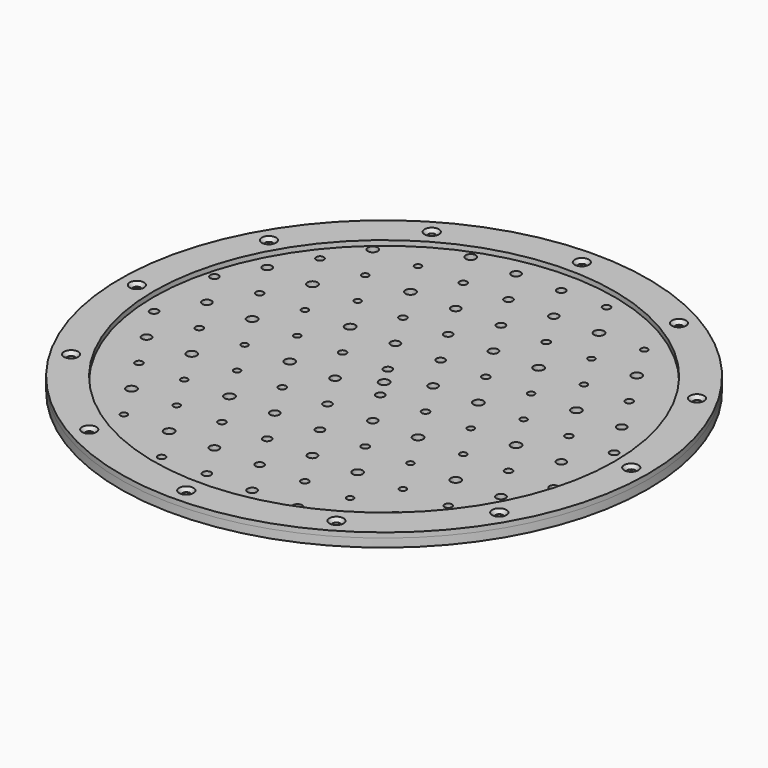
from build123d import *

# Parameters (mm, degrees)
F0_R     = 2.25
F0_R_2   = 2
F0_R_3   = 3
F0_R_4   = 2.75
F0_R_5   = 2.5
F1_DEPTH = 5
F2_R     = 157.5
F2_R_2   = 2
F2_R_3   = 137.5
F3_DEPTH = 5
F4_R     = 157.5
F4_R_2   = 2.25
F4_R_3   = 137.5
F5_DEPTH = 3
F6_SIZE  = 2


# Not quite as in the source:
# - a feature names something its author has since deleted; it is built from what else it names


with BuildPart() as f1:
    # F0 (on Top) → F1 (new body)
    with BuildSketch(Plane.XY):
        with BuildLine():
            Line((47.25, 82.8640606254), (47.25, 75.5725751183))
            ThreePointArc((47.25, 75.5725751183), (114.75, 57.8640606254), (182.25, 75.5725751183))
            ThreePointArc((182.25, 75.5725751183), (233.4671007058, 125.9918759979), (252.25, 195.3640606254))
            ThreePointArc((252.25, 195.3640606254), (233.4671007058, 264.736245253), (182.25, 315.1555461325))
            ThreePointArc((182.25, 315.1555461325), (114.75, 332.8640606254), (47.25, 315.1555461325))
            ThreePointArc((47.25, 315.1555461325), (-22.580141759, 202.1964953641), (35.6930584958, 82.8640606254))
            Line((35.6930584958, 82.8640606254), (47.25, 82.8640606254))
        make_face()
        with Locations((81, 71.6140606254)):
            Circle(F0_R, mode=Mode.SUBTRACT)
        with Locations((40.5, 94.1140606254)):
            Circle(F0_R_2, mode=Mode.SUBTRACT)
        with Locations((27, 116.6140606254)):
            Circle(F0_R_3, mode=Mode.SUBTRACT)
        with Locations((67.5, 94.1140606254)):
            Circle(F0_R_3, mode=Mode.SUBTRACT)
        with Locations((54, 116.6140606254)):
            Circle(F0_R_2, mode=Mode.SUBTRACT)
        with Locations((81, 116.6140606254)):
            Circle(F0_R, mode=Mode.SUBTRACT)
        with Locations((13.5, 139.1140606254)):
            Circle(F0_R, mode=Mode.SUBTRACT)
        with Locations((40.5, 139.1140606254)):
            Circle(F0_R_2, mode=Mode.SUBTRACT)
        with Locations((0, 161.6140606254)):
            Circle(F0_R_4, mode=Mode.SUBTRACT)
        with Locations((27, 161.6140606254)):
            Circle(F0_R_3, mode=Mode.SUBTRACT)
        with Locations((67.5, 139.1140606254)):
            Circle(F0_R_3, mode=Mode.SUBTRACT)
        with Locations((54, 161.6140606254)):
            Circle(F0_R_2, mode=Mode.SUBTRACT)
        with Locations((81, 161.6140606254)):
            Circle(F0_R, mode=Mode.SUBTRACT)
        with Locations((108, 71.6140606254)):
            Circle(F0_R_5, mode=Mode.SUBTRACT)
        with Locations((135, 71.6140606254)):
            Circle(F0_R_4, mode=Mode.SUBTRACT)
        with Locations((162, 71.6140606254)):
            Circle(F0_R_3, mode=Mode.SUBTRACT)
        with Locations((94.5, 94.1140606254)):
            Circle(F0_R_4, mode=Mode.SUBTRACT)
        with Locations((121.5, 94.1140606254)):
            Circle(F0_R_5, mode=Mode.SUBTRACT)
        with Locations((108, 116.6140606254)):
            Circle(F0_R_5, mode=Mode.SUBTRACT)
        with Locations((148.5, 94.1140606254)):
            Circle(F0_R, mode=Mode.SUBTRACT)
        with Locations((135, 116.6140606254)):
            Circle(F0_R_4, mode=Mode.SUBTRACT)
        with Locations((162, 116.6140606254)):
            Circle(F0_R_3, mode=Mode.SUBTRACT)
        with Locations((94.5, 139.1140606254)):
            Circle(F0_R_4, mode=Mode.SUBTRACT)
        with Locations((121.5, 139.1140606254)):
            Circle(F0_R_5, mode=Mode.SUBTRACT)
        with Locations((108, 161.6140606254)):
            Circle(F0_R_5, mode=Mode.SUBTRACT)
        with Locations((148.5, 139.1140606254)):
            Circle(F0_R, mode=Mode.SUBTRACT)
        with Locations((135, 161.6140606254)):
            Circle(F0_R_4, mode=Mode.SUBTRACT)
        with Locations((162, 161.6140606254)):
            Circle(F0_R_3, mode=Mode.SUBTRACT)
        with Locations((175.5, 94.1140606254)):
            Circle(F0_R_2, mode=Mode.SUBTRACT)
        with Locations((202.5, 94.1140606254)):
            Circle(F0_R_3, mode=Mode.SUBTRACT)
        with Locations((189, 116.6140606254)):
            Circle(F0_R_2, mode=Mode.SUBTRACT)
        with Locations((216, 116.6140606254)):
            Circle(F0_R, mode=Mode.SUBTRACT)
        with Locations((175.5, 139.1140606254)):
            Circle(F0_R_2, mode=Mode.SUBTRACT)
        with Locations((202.5, 139.1140606254)):
            Circle(F0_R_3, mode=Mode.SUBTRACT)
        with Locations((189, 161.6140606254)):
            Circle(F0_R_2, mode=Mode.SUBTRACT)
        with Locations((229.5, 139.1140606254)):
            Circle(F0_R_4, mode=Mode.SUBTRACT)
        with Locations((216, 161.6140606254)):
            Circle(F0_R, mode=Mode.SUBTRACT)
        with Locations((243, 161.6140606254)):
            Circle(F0_R_5, mode=Mode.SUBTRACT)
        with Locations((-13.5, 184.1140606254)):
            Circle(F0_R_5, mode=Mode.SUBTRACT)
        with Locations((-13.5, 229.1140606254)):
            Circle(F0_R_5, mode=Mode.SUBTRACT)
        with Locations((13.5, 184.1140606254)):
            Circle(F0_R, mode=Mode.SUBTRACT)
        with Locations((40.5, 184.1140606254)):
            Circle(F0_R_2, mode=Mode.SUBTRACT)
        with Locations((0, 206.6140606254)):
            Circle(F0_R_4, mode=Mode.SUBTRACT)
        with Locations((27, 206.6140606254)):
            Circle(F0_R_3, mode=Mode.SUBTRACT)
        with Locations((67.5, 184.1140606254)):
            Circle(F0_R_3, mode=Mode.SUBTRACT)
        with Locations((54, 206.6140606254)):
            Circle(F0_R_2, mode=Mode.SUBTRACT)
        with Locations((81, 206.6140606254)):
            Circle(F0_R, mode=Mode.SUBTRACT)
        with Locations((13.5, 229.1140606254)):
            Circle(F0_R, mode=Mode.SUBTRACT)
        with Locations((40.5, 229.1140606254)):
            Circle(F0_R_2, mode=Mode.SUBTRACT)
        with Locations((0, 251.6140606254)):
            Circle(F0_R_4, mode=Mode.SUBTRACT)
        with Locations((27, 251.6140606254)):
            Circle(F0_R_3, mode=Mode.SUBTRACT)
        with Locations((67.5, 229.1140606254)):
            Circle(F0_R_3, mode=Mode.SUBTRACT)
        with Locations((54, 251.6140606254)):
            Circle(F0_R_2, mode=Mode.SUBTRACT)
        with Locations((81, 251.6140606254)):
            Circle(F0_R, mode=Mode.SUBTRACT)
        with Locations((13.5, 274.1140606254)):
            Circle(F0_R, mode=Mode.SUBTRACT)
        with Locations((40.5, 274.1140606254)):
            Circle(F0_R_2, mode=Mode.SUBTRACT)
        with Locations((27, 296.6140606254)):
            Circle(F0_R_3, mode=Mode.SUBTRACT)
        with Locations((67.5, 274.1140606254)):
            Circle(F0_R_3, mode=Mode.SUBTRACT)
        with Locations((54, 296.6140606254)):
            Circle(F0_R_2, mode=Mode.SUBTRACT)
        with Locations((81, 296.6140606254)):
            Circle(F0_R, mode=Mode.SUBTRACT)
        with Locations((67.5, 319.1140606254)):
            Circle(F0_R_3, mode=Mode.SUBTRACT)
        with Locations((94.5, 184.1140606254)):
            Circle(F0_R_4, mode=Mode.SUBTRACT)
        with Locations((121.5, 184.1140606254)):
            Circle(F0_R_5, mode=Mode.SUBTRACT)
        with Locations((114.8160025477, 195.3414678574)):
            Circle(F0_R_3, mode=Mode.SUBTRACT)
        with Locations((108, 206.6140606254)):
            Circle(F0_R_5, mode=Mode.SUBTRACT)
        with Locations((148.5, 184.1140606254)):
            Circle(F0_R, mode=Mode.SUBTRACT)
        with Locations((135, 206.6140606254)):
            Circle(F0_R_4, mode=Mode.SUBTRACT)
        with Locations((162, 206.6140606254)):
            Circle(F0_R_3, mode=Mode.SUBTRACT)
        with Locations((94.5, 229.1140606254)):
            Circle(F0_R_4, mode=Mode.SUBTRACT)
        with Locations((121.5, 229.1140606254)):
            Circle(F0_R_5, mode=Mode.SUBTRACT)
        with Locations((108, 251.6140606254)):
            Circle(F0_R_5, mode=Mode.SUBTRACT)
        with Locations((148.5, 229.1140606254)):
            Circle(F0_R, mode=Mode.SUBTRACT)
        with Locations((135, 251.6140606254)):
            Circle(F0_R_4, mode=Mode.SUBTRACT)
        with Locations((162, 251.6140606254)):
            Circle(F0_R_3, mode=Mode.SUBTRACT)
        with Locations((175.5, 184.1140606254)):
            Circle(F0_R_2, mode=Mode.SUBTRACT)
        with Locations((202.5, 184.1140606254)):
            Circle(F0_R_3, mode=Mode.SUBTRACT)
        with Locations((189, 206.6140606254)):
            Circle(F0_R_2, mode=Mode.SUBTRACT)
        with Locations((229.5, 184.1140606254)):
            Circle(F0_R_4, mode=Mode.SUBTRACT)
        with Locations((216, 206.6140606254)):
            Circle(F0_R, mode=Mode.SUBTRACT)
        with Locations((243, 206.6140606254)):
            Circle(F0_R_5, mode=Mode.SUBTRACT)
        with Locations((175.5, 229.1140606254)):
            Circle(F0_R_2, mode=Mode.SUBTRACT)
        with Locations((202.5, 229.1140606254)):
            Circle(F0_R_3, mode=Mode.SUBTRACT)
        with Locations((189, 251.6140606254)):
            Circle(F0_R_2, mode=Mode.SUBTRACT)
        with Locations((229.5, 229.1140606254)):
            Circle(F0_R_4, mode=Mode.SUBTRACT)
        with Locations((216, 251.6140606254)):
            Circle(F0_R, mode=Mode.SUBTRACT)
        with Locations((94.5, 274.1140606254)):
            Circle(F0_R_4, mode=Mode.SUBTRACT)
        with Locations((121.5, 274.1140606254)):
            Circle(F0_R_5, mode=Mode.SUBTRACT)
        with Locations((108, 296.6140606254)):
            Circle(F0_R_5, mode=Mode.SUBTRACT)
        with Locations((148.5, 274.1140606254)):
            Circle(F0_R, mode=Mode.SUBTRACT)
        with Locations((135, 296.6140606254)):
            Circle(F0_R_4, mode=Mode.SUBTRACT)
        with Locations((162, 296.6140606254)):
            Circle(F0_R_3, mode=Mode.SUBTRACT)
        with Locations((94.5, 319.1140606254)):
            Circle(F0_R_4, mode=Mode.SUBTRACT)
        with Locations((121.5, 319.1140606254)):
            Circle(F0_R_5, mode=Mode.SUBTRACT)
        with Locations((148.5, 319.1140606254)):
            Circle(F0_R, mode=Mode.SUBTRACT)
        with Locations((175.5, 274.1140606254)):
            Circle(F0_R_2, mode=Mode.SUBTRACT)
        with Locations((202.5, 274.1140606254)):
            Circle(F0_R_3, mode=Mode.SUBTRACT)
        with Locations((189, 296.6140606254)):
            Circle(F0_R_2, mode=Mode.SUBTRACT)
        with BuildLine():
            ThreePointArc((35.6930584958, 82.8640606254), (41.3808939949, 79.0746617792), (47.25, 75.5725751183))
            Line((47.25, 75.5725751183), (47.25, 82.8640606254))
            Line((47.25, 82.8640606254), (35.6930584958, 82.8640606254))
        make_face()
    extrude(amount=F1_DEPTH)



with BuildPart() as f1b:
    # F0 (on Top) → F1, piece 2 (new body)
    with BuildSketch(Plane.XY):
        with Locations((40.5, 319.1140606254)):
            Circle(F0_R_2)
    extrude(amount=F1_DEPTH)


with BuildPart() as f1c:
    # F0 (on Top) → F1, piece 3 (new body)
    with BuildSketch(Plane.XY):
        with Locations((189, 71.6140606254)):
            Circle(F0_R_2)
    extrude(amount=F1_DEPTH)


with BuildPart() as f1_1:
    add(f1.part)

    add(f1b.part)  # F3 merges F1b

    add(f1c.part)  # F3 merges F1c
    # F2 (on Top) → F3 (join)
    with BuildSketch(Plane.XY):
        with Locations((114.75, 195.3640606254)):
            Circle(F2_R)
        with Locations((41, 67.6253135672)):
            Circle(F2_R_2, mode=Mode.SUBTRACT)
        with Locations((-12.9887470582, 121.6140606254)):
            Circle(F2_R_2, mode=Mode.SUBTRACT)
        with Locations((114.75, 47.8640606254)):
            Circle(F2_R_2, mode=Mode.SUBTRACT)
        with Locations((188.5, 67.6253135672)):
            Circle(F2_R_2, mode=Mode.SUBTRACT)
        with Locations((242.4887470582, 121.6140606254)):
            Circle(F2_R_2, mode=Mode.SUBTRACT)
        with Locations((-32.75, 195.3640606254)):
            Circle(F2_R_2, mode=Mode.SUBTRACT)
        with Locations((-12.9887470582, 269.1140606254)):
            Circle(F2_R_2, mode=Mode.SUBTRACT)
        with Locations((41, 323.1028076836)):
            Circle(F2_R_2, mode=Mode.SUBTRACT)
        with Locations((114.75, 195.3640606254)):
            Circle(F2_R_3, mode=Mode.SUBTRACT)
        with Locations((262.25, 195.3640606254)):
            Circle(F2_R_2, mode=Mode.SUBTRACT)
        with Locations((242.4887470582, 269.1140606254)):
            Circle(F2_R_2, mode=Mode.SUBTRACT)
        with Locations((114.75, 342.8640606254)):
            Circle(F2_R_2, mode=Mode.SUBTRACT)
        with Locations((188.5, 323.1028076836)):
            Circle(F2_R_2, mode=Mode.SUBTRACT)
    extrude(amount=F3_DEPTH)


with BuildPart() as f5:
    # F4 (on face) → F5 (new body)
    with BuildSketch(Plane.XY.offset(5)):
        with Locations((114.75, 195.3640606254)):
            Circle(F4_R)
        with Locations((41, 67.6253135672)):
            Circle(F4_R_2, mode=Mode.SUBTRACT)
        with Locations((-12.9887470582, 121.6140606254)):
            Circle(F4_R_2, mode=Mode.SUBTRACT)
        with Locations((114.75, 47.8640606254)):
            Circle(F4_R_2, mode=Mode.SUBTRACT)
        with Locations((188.5, 67.6253135672)):
            Circle(F4_R_2, mode=Mode.SUBTRACT)
        with Locations((242.4887470582, 121.6140606254)):
            Circle(F4_R_2, mode=Mode.SUBTRACT)
        with Locations((-32.75, 195.3640606254)):
            Circle(F4_R_2, mode=Mode.SUBTRACT)
        with Locations((-12.9887470582, 269.1140606254)):
            Circle(F4_R_2, mode=Mode.SUBTRACT)
        with Locations((41, 323.1028076836)):
            Circle(F4_R_2, mode=Mode.SUBTRACT)
        with Locations((114.75, 195.3640606254)):
            Circle(F4_R_3, mode=Mode.SUBTRACT)
        with Locations((262.25, 195.3640606254)):
            Circle(F4_R_2, mode=Mode.SUBTRACT)
        with Locations((242.4887470582, 269.1140606254)):
            Circle(F4_R_2, mode=Mode.SUBTRACT)
        with Locations((114.75, 342.8640606254)):
            Circle(F4_R_2, mode=Mode.SUBTRACT)
        with Locations((188.5, 323.1028076836)):
            Circle(F4_R_2, mode=Mode.SUBTRACT)
    extrude(amount=F5_DEPTH)

    # F6
    f6_edges = [f5.edges().sort_by_distance(p)[0] for p in [
        (112.5, 342.864061, 8),
        (186.25, 323.102808, 8),
        (240.238747, 269.114061, 8),
        (260, 195.364061, 8),
        (240.238747, 121.614061, 8),
        (38.75, 323.102808, 8),
        (-15.238747, 269.114061, 8),
        (-35, 195.364061, 8),
        (-15.238747, 121.614061, 8),
        (38.75, 67.625314, 8),
        (112.5, 47.864061, 8),
        (186.25, 67.625314, 8),
    ]]
    chamfer(f6_edges, length=F6_SIZE)


solid = Compound([f1_1.part, f5.part])
